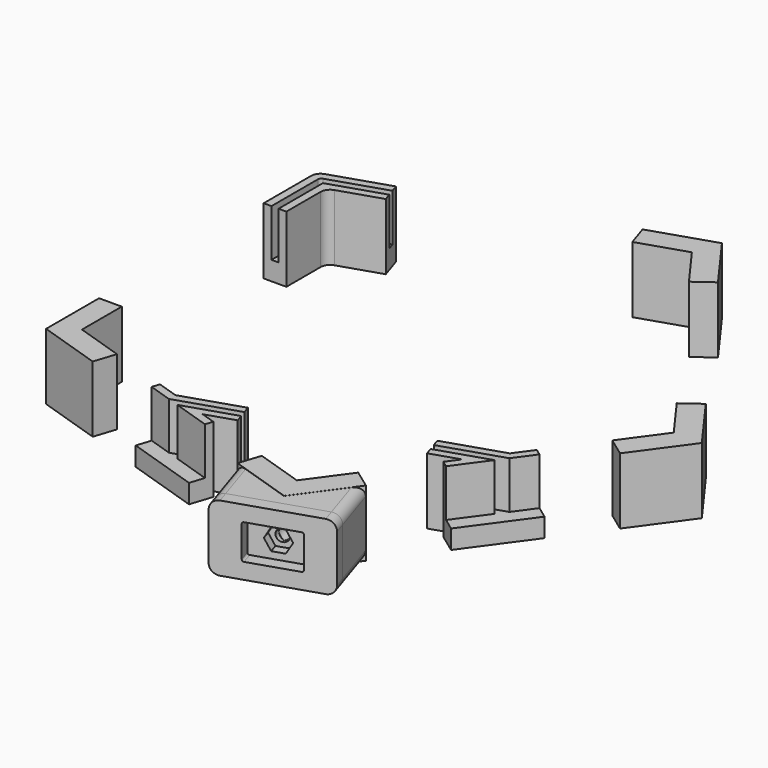
from build123d import *

# Parameters (mm, degrees)
F1_DEPTH  = 35
F3_DEPTH  = 25
F4_R      = 5
F6_DEPTH  = 25
F8_DEPTH  = 25
F9_R      = 5
F12_DEPTH = 5
F11_R     = 3.25
F13_DEPTH = 15
F14_W     = 40
F14_H     = 25
F15_DEPTH = 4.5
F16_W     = 40
F16_H     = 25
F17_DEPTH = 4.5
F18_DEPTH = 6.6
F20_DEPTH = 25


with BuildPart() as f1:
    # F0 (on Top) → F1 (new body)
    with BuildSketch(Plane.XY):
        Polygon((-89.7054851697, 100.1748499712), (-122.99246324, 89.359255168), (-122.99246324, 54.359255168), (-110.99246324, 54.359255168), (-110.99246324, 80.640744832), (-85.9972812372, 88.7621717756), align=None)
    extrude(amount=F1_DEPTH)


with BuildPart() as f1b:
    # F0 (on Top) → F1, piece 2 (new body)
    with BuildSketch(Plane.XY):
        Polygon((-89.7054851697, -100.1748499712), (-85.9972812372, -88.7621717756), (-110.99246324, -80.640744832), (-110.99246324, -54.359255168), (-122.99246324, -54.359255168), (-122.99246324, -89.359255168), align=None)
    extrude(amount=F1_DEPTH)


with BuildPart() as f1c:
    # F0 (on Top) → F1, piece 3 (new body)
    with BuildSketch(Plane.XY):
        Polygon((54.3953484626, -134.378502371), (67.5514244279, -116.2707172681), (57.8432204954, -109.2172942406), (42.3953484626, -130.4794660162), (17.4001664598, -122.3580390726), (13.6919625273, -133.7707172681), (46.9789405976, -144.5863120713), align=None)
    extrude(amount=F1_DEPTH)


with BuildPart() as f1d:
    # F0 (on Top) → F1, piece 4 (new body)
    with BuildSketch(Plane.XY):
        Polygon((131.4545614546, 28.3155948031), (121.7463575221, 21.2621717756), (137.1942295548, 0), (121.7463575221, -21.2621717756), (131.4545614546, -28.3155948031), (152.0270452848, 0), align=None)
    extrude(amount=F1_DEPTH)


with BuildPart() as f1e:
    # F0 (on Top) → F1, piece 5 (new body)
    with BuildSketch(Plane.XY):
        Polygon((67.5514244279, 116.2707172681), (46.9789405976, 144.5863120713), (13.6919625273, 133.7707172681), (17.4001664598, 122.3580390726), (42.3953484626, 130.4794660162), (57.8432204954, 109.2172942406), align=None)
    extrude(amount=F1_DEPTH)


with BuildPart() as f1f:
    # F0 (on Top) → F1, piece 6 (new body)
    with BuildSketch(Plane.XY):
        Polygon((-58.9940718149, -110.1535930693), (-20.9518111631, -122.5142728443), (-17.2436072306, -111.1015946487), (-24.8883169861, -108.6176778772), (-10.1627123972, -103.8330389073), (-13.8709163297, -92.4203607118), (-44.3047248511, -102.3089045318), (-55.2858678824, -98.7409148737), align=None)
    extrude(amount=F1_DEPTH)


with BuildPart() as f1g:
    # F0 (on Top) → F1, piece 7 (new body)
    with BuildSketch(Plane.XY):
        Polygon((112.4738641588, -54.440283399), (102.7656602263, -47.3868603715), (95.9789405976, -56.7279785677), (65.5451320762, -66.6165223877), (69.2533360087, -78.0292005833), (83.9789405976, -73.2445616134), (79.2542501346, -79.7475401465), (88.9624540671, -86.800963174), align=None)
    extrude(amount=F1_DEPTH)


with BuildPart() as f1h:
    # F0 (on Top) → F1, piece 8 (new body)
    with BuildSketch(Plane.XY):
        Polygon((13.7301591284, -133.8882743186), (22.0836515011, -159.5976802719), (75.9431134017, -142.0976802719), (67.589621029, -116.3882743186), (47.0171371988, -144.7038691217), align=None)
    extrude(amount=F1_DEPTH)

    # F9
    f9_edges = [f1h.edges().sort_by_distance(p)[0] for p in [
        (17.906905, -146.742977, 0),
        (17.906905, -146.742977, 35),
        (71.766367, -129.242977, 35),
        (71.766367, -129.242977, 0),
    ]]
    fillet(f9_edges, radius=F9_R)

    # F10 (on face) → F12 (cut)
    with BuildSketch(Plane(origin=(49.0133824514, -150.8476802719, 0), x_dir=(0.9510565163, 0.3090169944, 0), z_dir=(0.3090169944, -0.9510565163, 0))):
        Polygon((3.2331615075, 23.1), (-3.2331615075, 23.1), (-6.4663230149, 17.5), (-3.2331615075, 11.9), (3.2331615075, 11.9), (6.4663230149, 17.5), align=None)
    extrude(amount=-F12_DEPTH, mode=Mode.SUBTRACT)


with BuildPart() as f3_tool:
    # F2 (on face) → F3 (new body)
    with BuildSketch(Plane.XY.offset(35)):
        with BuildLine():
            Line((-38.2370973933, -108.6176778772), (-41.2709111222, -109.6034237124))
            Line((-41.2709111222, -109.6034237124), (-43.7253179867, -110.4009088452))
            ThreePointArc((-43.7253179867, -110.4009088452), (-44.3047247368, -110.4926778772), (-44.8841314982, -110.4009089159))
            Line((-44.8841314982, -110.4009089159), (-1.672213686, -124.441312125))
            ThreePointArc((-1.672213686, -124.441312125), (0.6904241465, -123.2374880214), (-0.5133999571, -120.8748501889))
            Line((-0.5133999571, -120.8748501889), (-38.2370973933, -108.6176778772))
        make_face()
        with BuildLine():
            ThreePointArc((-44.8841314982, -110.4009089159), (-45.9753620321, -109.468910166), (-46.0879558192, -108.0382710127))
            ThreePointArc((-46.0879558192, -108.0382710127), (-45.6305500658, -107.2918526625), (-44.8841317156, -106.8344469091))
            Line((-44.8841317156, -106.8344469091), (-44.3047248511, -106.6461862067))
            Line((-44.3047248511, -106.6461862067), (-66.3806738585, -99.4732755612))
            ThreePointArc((-66.3806738585, -99.4732755612), (-68.743311691, -100.6770996648), (-67.5394875874, -103.0397374973))
            Line((-67.5394875874, -103.0397374973), (-44.8841314982, -110.4009089159))
        make_face()
        with BuildLine():
            Line((111.5647467268, -42.2938259644), (98.5283308012, -60.2369131522))
            Line((98.5283308012, -60.2369131522), (99.1077376657, -60.0486524498))
            ThreePointArc((99.1077376657, -60.0486524498), (99.9804591521, -59.9799677792), (100.7892418782, -60.3149765534))
            ThreePointArc((100.7892418782, -60.3149765534), (101.5390601695, -61.5385688005), (101.2040513891, -62.9339807735))
            Line((101.2040513891, -62.9339807735), (114.5985604557, -44.4980206605))
            ThreePointArc((114.5985604557, -44.4980206605), (114.1837509393, -41.879016448), (111.5647467268, -42.2938259644))
        make_face()
        with BuildLine():
            Line((97.8121445301, -64.4125995187), (94.7783308012, -65.3983453539))
            Line((94.7783308012, -65.3983453539), (75.5809337275, -91.8212956063))
            ThreePointArc((75.5809337275, -91.8212956063), (75.9957432439, -94.4402998188), (78.6147474564, -94.0254903024))
            Line((78.6147474564, -94.0254903024), (101.2040513891, -62.9339807735))
            ThreePointArc((101.2040513891, -62.9339807735), (100.7892418744, -63.348790285), (100.2665513946, -63.6151143859))
            Line((100.2665513946, -63.6151143859), (97.8121445301, -64.4125995187))
        make_face()
        with BuildLine():
            Line((-116.99246324, 85), (-116.99246324, 83.125))
            ThreePointArc((-116.99246324, 83.125), (-116.6991486181, 83.1480843614), (-116.4130563756, 83.2167690319))
            Line((-116.4130563756, 83.2167690319), (-115.11746324, 83.63773276))
            Line((-115.11746324, 83.63773276), (-115.11746324, 85))
            ThreePointArc((-115.11746324, 85), (-115.1405476014, 85.293314622), (-115.209232272, 85.5794068645))
            Line((-115.209232272, 85.5794068645), (-116.99246324, 85))
        make_face()
        Polygon((-44.3047248511, -106.6461862067), (-41.2709111222, -107.631932042), (96.6533308012, -62.8176292531), (98.5283308012, -60.2369131522), align=None)
        with BuildLine():
            ThreePointArc((-118.86746324, 85), (-118.3182884548, 83.6741747853), (-116.99246324, 83.125))
            Line((-116.99246324, 83.125), (-116.99246324, 85))
            Line((-116.99246324, 85), (-115.209232272, 85.5794068645))
            ThreePointArc((-115.209232272, 85.5794068645), (-116.141231053, 86.6706372329), (-117.5718701045, 86.7832309681))
            ThreePointArc((-117.5718701045, 86.7832309681), (-118.5093701045, 86.102097348), (-118.86746324, 85))
        make_face()
        with BuildLine():
            Line((-46.0879558192, -108.0382710127), (-44.3047248511, -108.6176778772))
            Line((-44.3047248511, -108.6176778772), (-41.2709111222, -107.631932042))
            Line((-41.2709111222, -107.631932042), (-44.3047248511, -106.6461862067))
            Line((-44.3047248511, -106.6461862067), (-44.8841317156, -106.8344469091))
            ThreePointArc((-44.8841317156, -106.8344469091), (-45.6305500658, -107.2918526625), (-46.0879558192, -108.0382710127))
        make_face()
        Polygon((-41.2709111222, -107.631932042), (-44.3047248511, -108.6176778772), (-41.2709111222, -109.6034237124), (-38.2370973933, -108.6176778772), align=None)
        with BuildLine():
            Line((98.5283308012, -60.2369131522), (96.6533308012, -62.8176292531))
            Line((96.6533308012, -62.8176292531), (99.6871445301, -61.8318834178))
            Line((99.6871445301, -61.8318834178), (100.7892418782, -60.3149765534))
            ThreePointArc((100.7892418782, -60.3149765534), (99.9804591521, -59.9799677792), (99.1077376657, -60.0486524498))
            Line((99.1077376657, -60.0486524498), (98.5283308012, -60.2369131522))
        make_face()
        Polygon((99.6871445301, -61.8318834178), (96.6533308012, -62.8176292531), (94.7783308012, -65.3983453539), (97.8121445301, -64.4125995187), align=None)
        with BuildLine():
            Line((100.7892418782, -60.3149765534), (99.6871445301, -61.8318834178))
            Line((99.6871445301, -61.8318834178), (97.8121445301, -64.4125995187))
            Line((97.8121445301, -64.4125995187), (100.2665513946, -63.6151143859))
            ThreePointArc((100.2665513946, -63.6151143859), (100.7892418744, -63.348790285), (101.2040513891, -62.9339807735))
            ThreePointArc((101.2040513891, -62.9339807735), (101.5390601695, -61.5385688005), (100.7892418782, -60.3149765534))
        make_face()
        with BuildLine():
            Line((-41.2709111222, -109.6034237124), (-44.3047248511, -108.6176778772))
            Line((-44.3047248511, -108.6176778772), (-46.0879558192, -108.0382710127))
            ThreePointArc((-46.0879558192, -108.0382710127), (-45.9753620321, -109.468910166), (-44.8841314982, -110.4009089159))
            ThreePointArc((-44.8841314982, -110.4009089159), (-44.3047247368, -110.4926778772), (-43.7253179867, -110.4009088452))
            Line((-43.7253179867, -110.4009088452), (-41.2709111222, -109.6034237124))
        make_face()
        with BuildLine():
            Line((-118.86746324, 54.359255168), (-116.99246324, 54.359255168))
            Line((-116.99246324, 54.359255168), (-116.99246324, 83.125))
            ThreePointArc((-116.99246324, 83.125), (-118.3182884548, 83.6741747853), (-118.86746324, 85))
            Line((-118.86746324, 85), (-118.86746324, 54.359255168))
        make_face()
        with BuildLine():
            Line((-116.99246324, 83.125), (-116.99246324, 54.359255168))
            Line((-116.99246324, 54.359255168), (-115.11746324, 54.359255168))
            Line((-115.11746324, 54.359255168), (-115.11746324, 83.63773276))
            Line((-115.11746324, 83.63773276), (-116.4130563756, 83.2167690319))
            ThreePointArc((-116.4130563756, 83.2167690319), (-116.6991486181, 83.1480843614), (-116.99246324, 83.125))
        make_face()
        with BuildLine():
            ThreePointArc((-117.5718701045, 86.7832309681), (-116.141231053, 86.6706372329), (-115.209232272, 85.5794068645))
            Line((-115.209232272, 85.5794068645), (-87.8513832035, 94.4685108734))
            Line((-87.8513832035, 94.4685108734), (-88.4307900679, 96.2517418414))
            Line((-88.4307900679, 96.2517418414), (-117.5718701045, 86.7832309681))
        make_face()
        with BuildLine():
            Line((-115.11746324, 85), (-115.11746324, 83.63773276))
            Line((-115.11746324, 83.63773276), (-87.271976339, 92.6852799053))
            Line((-87.271976339, 92.6852799053), (-87.8513832035, 94.4685108734))
            Line((-87.8513832035, 94.4685108734), (-115.209232272, 85.5794068645))
            ThreePointArc((-115.209232272, 85.5794068645), (-115.1405476014, 85.293314622), (-115.11746324, 85))
        make_face()
        with BuildLine():
            Line((-115.11746324, 54.359255168), (-116.99246324, 54.359255168))
            Line((-116.99246324, 54.359255168), (-118.86746324, 54.359255168))
            ThreePointArc((-118.86746324, 54.359255168), (-116.99246324, 52.484255168), (-115.11746324, 54.359255168))
        make_face()
        with BuildLine():
            Line((-87.8513832035, 94.4685108734), (-87.271976339, 92.6852799053))
            ThreePointArc((-87.271976339, 92.6852799053), (-86.0681522354, 95.0479177378), (-88.4307900679, 96.2517418414))
            Line((-88.4307900679, 96.2517418414), (-87.8513832035, 94.4685108734))
        make_face()
    extrude(amount=-F3_DEPTH)


with BuildPart() as f1_1:
    add(f1.part)

    # F3: cut by f3_tool
    add(f3_tool.part, mode=Mode.SUBTRACT)

    # F4
    f4_edges = [f1_1.edges().sort_by_distance(p)[0] for p in [
        (-110.992463, 80.640745, 17.5),
        (-122.992463, 89.359255, 17.5),
    ]]
    fillet(f4_edges, radius=F4_R)

    # F7 (on face) → F8 (cut)
    with BuildSketch(Plane.XY.offset(35)):
        with BuildLine():
            Line((97.8121445301, -64.4125995187), (94.7783308012, -65.3983453539))
            Line((94.7783308012, -65.3983453539), (82.5914452364, -82.1721543122))
            Line((82.5914452364, -82.1721543122), (75.6043512253, -91.7890641857))
            ThreePointArc((75.6043512253, -91.7890641857), (76.0191607417, -94.4080683982), (78.6381649542, -93.9932588818))
            Line((78.6381649542, -93.9932588818), (101.2040513891, -62.9339807735))
            ThreePointArc((101.2040513891, -62.9339807735), (100.7892418744, -63.348790285), (100.2665513946, -63.6151143859))
            Line((100.2665513946, -63.6151143859), (97.8121445301, -64.4125995187))
        make_face()
        Polygon((99.6871445301, -61.8318834178), (96.6533308012, -62.8176292531), (94.7783308012, -65.3983453539), (97.8121445301, -64.4125995187), align=None)
        Polygon((-44.5022110645, -106.7103533672), (-41.4683973356, -107.6960992024), (96.6533308012, -62.8176292531), (98.5283308012, -60.2369131522), align=None)
        with BuildLine():
            Line((98.5283308012, -60.2369131522), (96.6533308012, -62.8176292531))
            Line((96.6533308012, -62.8176292531), (99.6871445301, -61.8318834178))
            Line((99.6871445301, -61.8318834178), (100.7892418782, -60.3149765534))
            ThreePointArc((100.7892418782, -60.3149765534), (99.9804591521, -59.9799677792), (99.1077376657, -60.0486524498))
            Line((99.1077376657, -60.0486524498), (98.5283308012, -60.2369131522))
        make_face()
        with BuildLine():
            Line((111.5881642246, -42.2615945438), (98.5283308012, -60.2369131522))
            Line((98.5283308012, -60.2369131522), (99.1077376657, -60.0486524498))
            ThreePointArc((99.1077376657, -60.0486524498), (99.9804591521, -59.9799677792), (100.7892418782, -60.3149765534))
            ThreePointArc((100.7892418782, -60.3149765534), (101.5390601695, -61.5385688005), (101.2040513891, -62.9339807735))
            Line((101.2040513891, -62.9339807735), (114.6219779535, -44.4657892399))
            ThreePointArc((114.6219779535, -44.4657892399), (114.2071684371, -41.8467850274), (111.5881642246, -42.2615945438))
        make_face()
        with BuildLine():
            Line((100.7892418782, -60.3149765534), (99.6871445301, -61.8318834178))
            Line((99.6871445301, -61.8318834178), (97.8121445301, -64.4125995187))
            Line((97.8121445301, -64.4125995187), (100.2665513946, -63.6151143859))
            ThreePointArc((100.2665513946, -63.6151143859), (100.7892418744, -63.348790285), (101.2040513891, -62.9339807735))
            ThreePointArc((101.2040513891, -62.9339807735), (101.5390601695, -61.5385688005), (100.7892418782, -60.3149765534))
        make_face()
        Polygon((96.6533308012, -62.8176292531), (-41.4683973356, -107.6960992024), (-38.4345836067, -108.6818450377), (67.9786409069, -74.1060924535), (94.7783308012, -65.3983453539), align=None)
    extrude(amount=-F8_DEPTH, mode=Mode.SUBTRACT)


with BuildPart() as f1f_1:
    add(f1f.part)

    # F3: cut by f3_tool
    add(f3_tool.part, mode=Mode.SUBTRACT)


with BuildPart() as f1g_1:
    add(f1g.part)

    # F3: cut by f3_tool
    add(f3_tool.part, mode=Mode.SUBTRACT)


with BuildPart() as f6_tool:
    # F5 (on face) → F6 (new body)
    with BuildSketch(Plane.XY.offset(35)):
        with BuildLine():
            ThreePointArc((-44.8841315729, -110.4009088916), (-45.9753620499, -109.4689101311), (-46.0879558192, -108.0382710127))
            ThreePointArc((-46.0879558192, -108.0382710127), (-45.6305500658, -107.2918526625), (-44.8841317156, -106.8344469091))
            Line((-44.8841317156, -106.8344469091), (-44.3047248511, -106.6461862067))
            Line((-44.3047248511, -106.6461862067), (-66.8842523844, -99.3096529795))
            ThreePointArc((-66.8842523844, -99.3096529795), (-69.2468902169, -100.5134770831), (-68.0430661133, -102.8761149157))
            Line((-68.0430661133, -102.8761149157), (-44.8841315729, -110.4009088916))
        make_face()
        with BuildLine():
            Line((-41.2709111222, -109.6034237124), (-44.3047248511, -108.6176778772))
            Line((-44.3047248511, -108.6176778772), (-46.0879558192, -108.0382710127))
            ThreePointArc((-46.0879558192, -108.0382710127), (-45.9753620499, -109.4689101311), (-44.8841315729, -110.4009088916))
            ThreePointArc((-44.8841315729, -110.4009088916), (-44.3047247761, -110.4926778772), (-43.7253179867, -110.4009088452))
            Line((-43.7253179867, -110.4009088452), (-41.2709111222, -109.6034237124))
        make_face()
        with BuildLine():
            Line((-46.0879558192, -108.0382710127), (-44.3047248511, -108.6176778772))
            Line((-44.3047248511, -108.6176778772), (-41.2709111222, -107.631932042))
            Line((-41.2709111222, -107.631932042), (-44.3047248511, -106.6461862067))
            Line((-44.3047248511, -106.6461862067), (-44.8841317156, -106.8344469091))
            ThreePointArc((-44.8841317156, -106.8344469091), (-45.6305500658, -107.2918526625), (-46.0879558192, -108.0382710127))
        make_face()
        Polygon((-41.2709111222, -107.631932042), (-44.3047248511, -108.6176778772), (-41.2709111222, -109.6034237124), (-38.2370973933, -108.6176778772), align=None)
        Polygon((-44.3047248511, -106.6461862067), (-41.2709111222, -107.631932042), (-12.0168143634, -98.1266998095), (96.6533308012, -62.8176292531), (98.5283308012, -60.2369131522), align=None)
        Polygon((-12.0168143634, -98.1266998095), (-41.2709111222, -107.631932042), (-38.2370973933, -108.6176778772), (-11.437407499, -99.9099307776), align=None)
        with BuildLine():
            Line((-38.2370973933, -108.6176778772), (-41.2709111222, -109.6034237124))
            Line((-41.2709111222, -109.6034237124), (-43.7253179867, -110.4009088452))
            ThreePointArc((-43.7253179867, -110.4009088452), (-44.3047247761, -110.4926778772), (-44.8841315729, -110.4009088916))
            Line((-44.8841315729, -110.4009088916), (-2.1757922119, -124.2776895434))
            ThreePointArc((-2.1757922119, -124.2776895434), (0.1868456206, -123.0738654398), (-1.016978483, -120.7112276073))
            Line((-1.016978483, -120.7112276073), (-18.5183023324, -115.0247027784))
            Line((-18.5183023324, -115.0247027784), (-38.2370973933, -108.6176778772))
        make_face()
        Polygon((96.6533308012, -62.8176292531), (-12.0168143634, -98.1266998095), (-11.437407499, -99.9099307776), (94.7783308012, -65.3983453539), align=None)
        with BuildLine():
            Line((100.7892418782, -60.3149765534), (99.6871445301, -61.8318834178))
            Line((99.6871445301, -61.8318834178), (97.8121445301, -64.4125995187))
            Line((97.8121445301, -64.4125995187), (100.2665513946, -63.6151143859))
            ThreePointArc((100.2665513946, -63.6151143859), (100.7892419327, -63.3487902427), (101.2040514738, -62.9339806568))
            ThreePointArc((101.2040514738, -62.9339806568), (101.5390601582, -61.5385687293), (100.7892418782, -60.3149765534))
        make_face()
        with BuildLine():
            Line((98.5283308012, -60.2369131522), (96.6533308012, -62.8176292531))
            Line((96.6533308012, -62.8176292531), (99.6871445301, -61.8318834178))
            Line((99.6871445301, -61.8318834178), (100.7892418782, -60.3149765534))
            ThreePointArc((100.7892418782, -60.3149765534), (99.9804591521, -59.9799677792), (99.1077376657, -60.0486524498))
            Line((99.1077376657, -60.0486524498), (98.5283308012, -60.2369131522))
        make_face()
        Polygon((99.6871445301, -61.8318834178), (96.6533308012, -62.8176292531), (94.7783308012, -65.3983453539), (97.8121445301, -64.4125995187), align=None)
        with BuildLine():
            Line((97.8121445301, -64.4125995187), (94.7783308012, -65.3983453539))
            Line((94.7783308012, -65.3983453539), (75.4062468998, -92.0617313977))
            ThreePointArc((75.4062468998, -92.0617313977), (75.8210564162, -94.6807356102), (78.4400606287, -94.2659260938))
            Line((78.4400606287, -94.2659260938), (101.2040514738, -62.9339806568))
            ThreePointArc((101.2040514738, -62.9339806568), (100.7892419327, -63.3487902427), (100.2665513946, -63.6151143859))
            Line((100.2665513946, -63.6151143859), (97.8121445301, -64.4125995187))
        make_face()
        with BuildLine():
            Line((111.3900598991, -42.5342617558), (98.5283308012, -60.2369131522))
            Line((98.5283308012, -60.2369131522), (99.1077376657, -60.0486524498))
            ThreePointArc((99.1077376657, -60.0486524498), (99.9804591521, -59.9799677792), (100.7892418782, -60.3149765534))
            ThreePointArc((100.7892418782, -60.3149765534), (101.5390601582, -61.5385687293), (101.2040514738, -62.9339806568))
            Line((101.2040514738, -62.9339806568), (114.423873628, -44.7384564519))
            ThreePointArc((114.423873628, -44.7384564519), (114.0090641116, -42.1194522394), (111.3900598991, -42.5342617558))
        make_face()
    extrude(amount=-F6_DEPTH)


with BuildPart() as f1f_2:
    add(f1f_1.part)

    # F6: cut by f6_tool
    add(f6_tool.part, mode=Mode.SUBTRACT)

    # F14 (on face) → F15 (cut)
    with BuildSketch(Plane(origin=(-38.0067613212, -116.9727836196, 0), x_dir=(0.9510565163, -0.3090169944, 0), z_dir=(-0.3090169944, -0.9510565163, 0))):
        with Locations((-2.0673641725, 22.5)):
            Rectangle(F14_W, F14_H)
    extrude(amount=-F15_DEPTH, mode=Mode.SUBTRACT)


with BuildPart() as f1g_2:
    add(f1g_1.part)

    # F6: cut by f6_tool
    add(f6_tool.part, mode=Mode.SUBTRACT)

    # F16 (on face) → F17 (cut)
    with BuildSketch(Plane(origin=(99.5029929412, -72.2931560356, 0), x_dir=(0.5877852523, 0.8090169944, 0), z_dir=(0.8090169944, -0.5877852523, 0))):
        with Locations((2.0673641725, 22.5)):
            Rectangle(F16_W, F16_H)
    extrude(amount=-F17_DEPTH, mode=Mode.SUBTRACT)


with BuildPart() as f13_tool:
    # F11 (on face) → F13 (new body)
    with BuildSketch(Plane(origin=(49.0133824514, -150.8476802719, 0), x_dir=(0.9510565163, 0.3090169944, 0), z_dir=(0.3090169944, -0.9510565163, 0))):
        with Locations((0, 17.5)):
            Circle(F11_R)
    extrude(amount=-F13_DEPTH)


with BuildPart() as f1c_1:
    add(f1c.part)

    # F13: cut by f13_tool
    add(f13_tool.part, mode=Mode.SUBTRACT)


with BuildPart() as f1h_1:
    add(f1h.part)

    # F13: cut by f13_tool
    add(f13_tool.part, mode=Mode.SUBTRACT)


with BuildPart() as f18:
    # F18 (new): a face of the model
    f18_faces = [f1h_1.part.faces().sort_by_distance(p)[0] for p in [
        (22.7168074491, -159.3919554336, 17.5),
    ]]
    extrude(f18_faces, amount=F18_DEPTH)

    # F19 (on face) → F20 (cut)
    with BuildSketch(Plane(origin=(51.0528946143, -157.1246532794, 0), x_dir=(0.9510565163, 0.3090169944, 0), z_dir=(0.3090169944, -0.9510565163, 0))):
        with BuildLine():
            ThreePointArc((13.725, 25.8345645875), (13.4321067812, 26.5416713687), (12.725, 26.8345645875))
            Line((12.725, 26.8345645875), (-12.725, 26.8345645875))
            ThreePointArc((-12.725, 26.8345645875), (-13.4321067812, 26.5416713687), (-13.725, 25.8345645875))
            Line((-13.725, 25.8345645875), (-13.725, 9.3845645875))
            ThreePointArc((-13.725, 9.3845645875), (-13.4321067812, 8.6774578063), (-12.725, 8.3845645875))
            Line((-12.725, 8.3845645875), (12.725, 8.3845645875))
            ThreePointArc((12.725, 8.3845645875), (13.4321067812, 8.6774578063), (13.725, 9.3845645875))
            Line((13.725, 9.3845645875), (13.725, 25.8345645875))
        make_face()
    extrude(amount=-F20_DEPTH, mode=Mode.SUBTRACT)


solid = Compound([f1b.part, f1d.part, f1e.part, f1_1.part, f1f_2.part, f1g_2.part, f1c_1.part, f1h_1.part, f18.part])
